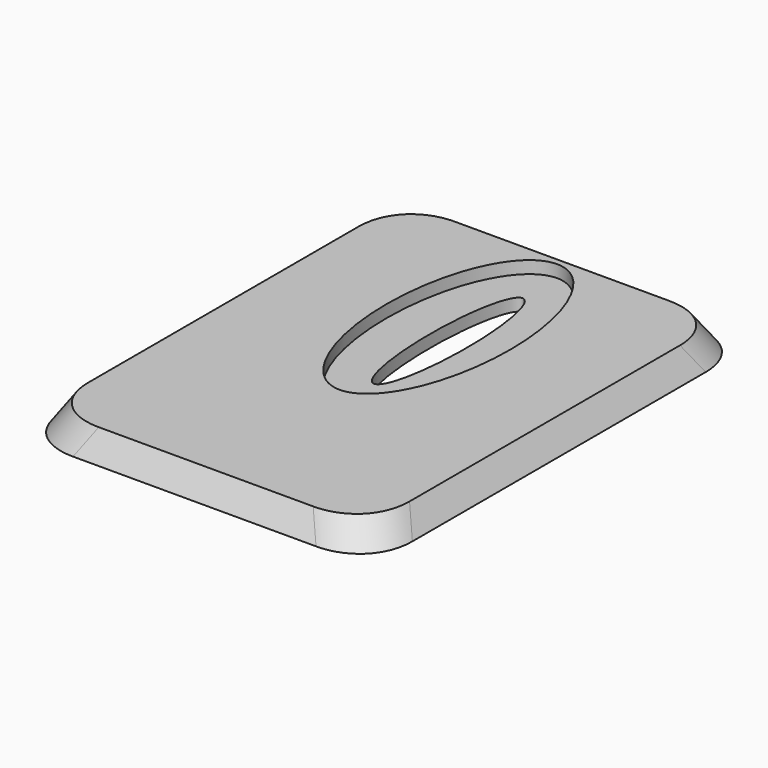
from build123d import *

# Parameters (mm, degrees)
F0_W        = 30
F0_H        = 40
F1_DEPTH    = 2
F3_DEPTH    = 1
F4_DEPTH    = 2
F5_T1_DEPTH = 47.9238558823
F5_T3_DEPTH = 57.9238558823
F6_R        = 5


# Not quite as in the source:
# - a fillet or chamfer that OpenCascade refuses, or shapes differently, is made with other operations: its cross-section is extruded or revolved along the edge and cut away or added


with BuildPart() as f1:
    # F0 (on Top) → F1 (new body)
    with BuildSketch(Plane.XY):
        with Locations((15, 20)):
            Rectangle(F0_W, F0_H)
    extrude(amount=F1_DEPTH)

    # F2 (on face) → F3 (cut)
    with BuildSketch(Plane.XY.offset(2)):
        with BuildLine():
            add(Edge.make_bspline(
                [(15, 37.5), (6.3397459622, 37.5), (10.6698729811, 21), (15, 4.5), (19.3301270189, 21), (23.6602540378, 37.5), (15, 37.5)],
                knots=[0, 0, 0, 2.0943951024, 2.0943951024, 4.1887902048, 4.1887902048, 6.2831853072, 6.2831853072, 6.2831853072], degree=2, weights=[1, 0.5, 1, 0.5, 1, 0.5, 1]))
        make_face()
        with BuildLine():
            add(Edge.make_bspline(
                [(15, 19), (17.5980762114, 19), (16.2990381057, 30.25), (15, 41.5), (13.7009618943, 30.25), (12.4019237886, 19), (15, 19)],
                knots=[0, 0, 0, 2.0943951024, 2.0943951024, 4.1887902048, 4.1887902048, 6.2831853072, 6.2831853072, 6.2831853072], degree=2, weights=[1, 0.5, 1, 0.5, 1, 0.5, 1]))
        make_face(mode=Mode.SUBTRACT)
    extrude(amount=-F3_DEPTH, mode=Mode.SUBTRACT)

    # F4 (cut): a face of the model
    f4_faces = [f1.faces().sort_by_distance(p)[0] for p in [
        (15, 26.5181913431, 2),
    ]]
    extrude(f4_faces, amount=-F4_DEPTH, mode=Mode.SUBTRACT)

    # F5: chamfer of 2 x 3.4641016151 on 4 edges, made by hand

    # F5_s2 → F5_t1 (cut)
    with BuildSketch(Plane.YZ.offset(-8.9619279412)):
        Polygon((0, -1.4641016151), (2, 2), (0, 2), align=None)
        Polygon((40, -1.4641016151), (38, 2), (40, 2), align=None)
    extrude(amount=F5_T1_DEPTH, mode=Mode.SUBTRACT)

    # F5_s4 → F5_t3 (cut)
    with BuildSketch(Plane.XZ.offset(-48.9619279412)):
        Polygon((28, 2), (30, -1.4641016151), (30, 2), align=None)
        Polygon((0, -1.4641016151), (2, 2), (0, 2), align=None)
    extrude(amount=F5_T3_DEPTH, mode=Mode.SUBTRACT)

    # F6
    f6_edges = [f1.edges().sort_by_distance(p)[0] for p in [
        (28.57735, 38.57735, 1),
        (28.57735, 1.42265, 1),
        (1.42265, 1.42265, 1),
        (1.42265, 38.57735, 1),
    ]]
    fillet(f6_edges, radius=F6_R)


solid = f1.part
